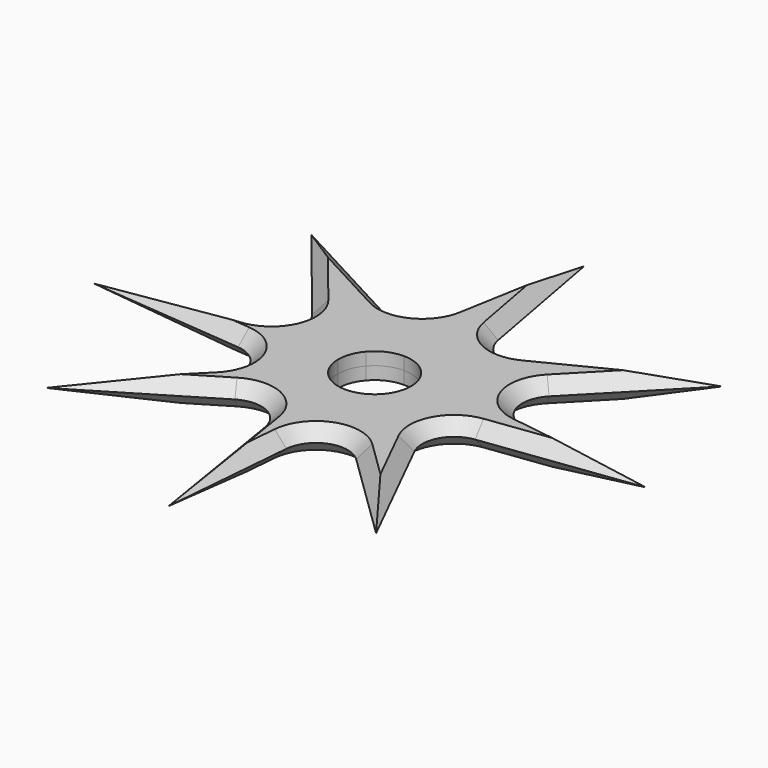
from build123d import *

# Parameters (mm, degrees)
F1_DEPTH = 2.54
F2_SIZE  = 2.53999


# Not quite as in the source:
# - a fillet or chamfer is up to 0.001 mm smaller than in the source, because OpenCascade refuses the exact size


with BuildPart() as f1:
    # F0 (on Top) → F1 (new body)
    with BuildSketch(Plane.XY):
        with BuildLine():
            ThreePointArc((-5.5453096033, 4.7335261172), (-3.0532951973, 6.6207338367), (0, 7.2908660733))
            Line((0, 7.2908660733), (0, 52.4203432724))
            Line((0, 52.4203432724), (-4.8945622179, 24.7540763342))
            ThreePointArc((-4.8945622179, 24.7540763342), (-8.3763552073, 20.1468586178), (-14.1500344693, 20.2650334375))
            Line((-14.1500344693, 20.2650334375), (-39.9762034536, 34.1240465641))
            Line((-39.9762034536, 34.1240465641), (-5.5453096033, 4.7335261172))
        make_face()
        with BuildLine():
            Line((0, 52.4203432724), (0, 7.2908660733))
            ThreePointArc((0, 7.2908660733), (3.1432479122, 6.5785044395), (5.6722672278, 4.5806236032))
            Line((5.6722672278, 4.5806236032), (42.2564104309, 34.1240465641))
            Line((42.2564104309, 34.1240465641), (14.255672391, 19.9525133065))
            ThreePointArc((14.255672391, 19.9525133065), (8.5682529825, 19.9287025413), (5.1430312406, 24.46909487))
            Line((5.1430312406, 24.46909487), (0, 52.4203432724))
        make_face()
        with BuildLine():
            ThreePointArc((5.6722672278, 4.5806236032), (6.8743170129, 2.4290931856), (7.2908660733, 0))
            ThreePointArc((7.2908660733, 0), (6.5785044395, -3.1432479122), (4.5806236032, -5.6722672278))
            Line((4.5806236032, -5.6722672278), (31.0746654868, -38.4803079069))
            Line((31.0746654868, -38.4803079069), (18.4844070176, -13.1473843843))
            ThreePointArc((18.4844070176, -13.1473843843), (18.5684546903, -7.3320030677), (23.3522337103, -4.024257286))
            Line((23.3522337103, -4.024257286), (54.3080642819, 0))
            Line((54.3080642819, 0), (26.9017063995, 3.9009043758))
            ThreePointArc((26.9017063995, 3.9009043758), (21.7859881354, 8.139124947), (23.2488130784, 14.6193433195))
            Line((23.2488130784, 14.6193433195), (42.2564104309, 34.1240465641))
            Line((42.2564104309, 34.1240465641), (5.6722672278, 4.5806236032))
        make_face()
        with BuildLine():
            ThreePointArc((4.5806236032, -5.6722672278), (2.4290931856, -6.8743170129), (0, -7.2908660733))
            Line((0, -7.2908660733), (0, -51.5490919352))
            Line((0, -51.5490919352), (2.255521124, -24.8929502638))
            ThreePointArc((2.255521124, -24.8929502638), (6.3641325232, -19.4785950158), (13.0147117735, -20.8806385306))
            Line((13.0147117735, -20.8806385306), (31.0746654868, -38.4803079069))
            Line((31.0746654868, -38.4803079069), (4.5806236032, -5.6722672278))
        make_face()
        with BuildLine():
            Line((0, -51.5490919352), (0, -7.2908660733))
            ThreePointArc((0, -7.2908660733), (-3.1432479122, -6.5785044395), (-5.6722672278, -4.5806236032))
            Line((-5.6722672278, -4.5806236032), (-39.9762034536, -32.2826717697))
            Line((-39.9762034536, -32.2826717697), (-14.4636689781, -16.8901939339))
            ThreePointArc((-14.4636689781, -16.8901939339), (-8.5166009917, -16.5643608756), (-4.9155814374, -21.3084564677))
            Line((-4.9155814374, -21.3084564677), (0, -51.5490919352))
        make_face()
        with BuildLine():
            ThreePointArc((-5.6722672278, -4.5806236032), (-6.8743170129, -2.4290931856), (-7.2908660733, 0))
            Line((-7.2908660733, 0), (-13.3722843602, 0))
            Line((-13.3722843602, 0), (-56.1868394799, 0))
            Line((-56.1868394799, 0), (-25.1595931562, -2.7541493308))
            ThreePointArc((-25.1595931562, -2.7541493308), (-19.7516975402, -6.9137834915), (-21.2347588093, -13.5732444768))
            Line((-21.2347588093, -13.5732444768), (-39.9762034536, -32.2826717697))
            Line((-39.9762034536, -32.2826717697), (-5.6722672278, -4.5806236032))
        make_face()
        with BuildLine():
            Line((-13.3722843602, 0), (-7.2908660733, 0))
            ThreePointArc((-7.2908660733, 0), (-6.8405715313, 2.5225600534), (-5.5453096033, 4.7335261172))
            Line((-5.5453096033, 4.7335261172), (-39.9762034536, 34.1240465641))
            Line((-39.9762034536, 34.1240465641), (-22.9918849286, 13.0920645237))
            ThreePointArc((-22.9918849286, 13.0920645237), (-22.0777388727, 6.6432422744), (-27.3229831249, 2.7818456164))
            Line((-27.3229831249, 2.7818456164), (-56.1868394799, 0))
            Line((-56.1868394799, 0), (-13.3722843602, 0))
        make_face()
    extrude(amount=F1_DEPTH)

    # F2 (size 2.54 in the source; OpenCascade refuses exactly that, so slightly less here)
    f2_edges = [f1.edges().sort_by_distance(p)[0] for p in [
        (28.256041, 27.03828, 2.54),
        (40.604885, 1.950452, 2.54),
        (24.779536, -25.813846, 2.54),
        (22.044689, -29.680473, 2.54),
        (-2.447281, 38.58721, 2.54),
        (-31.484044, 23.608056, 2.54),
        (-30.605481, -22.927958, 2.54),
        (-2.457791, -36.428774, 2.54),
    ]]
    chamfer(f2_edges, length=F2_SIZE)

    # F3: F1 across plane


with BuildPart() as f1_1:
    add(f1.part)
    add(f1.part.mirror(Plane.XY))


solid = f1_1.part
